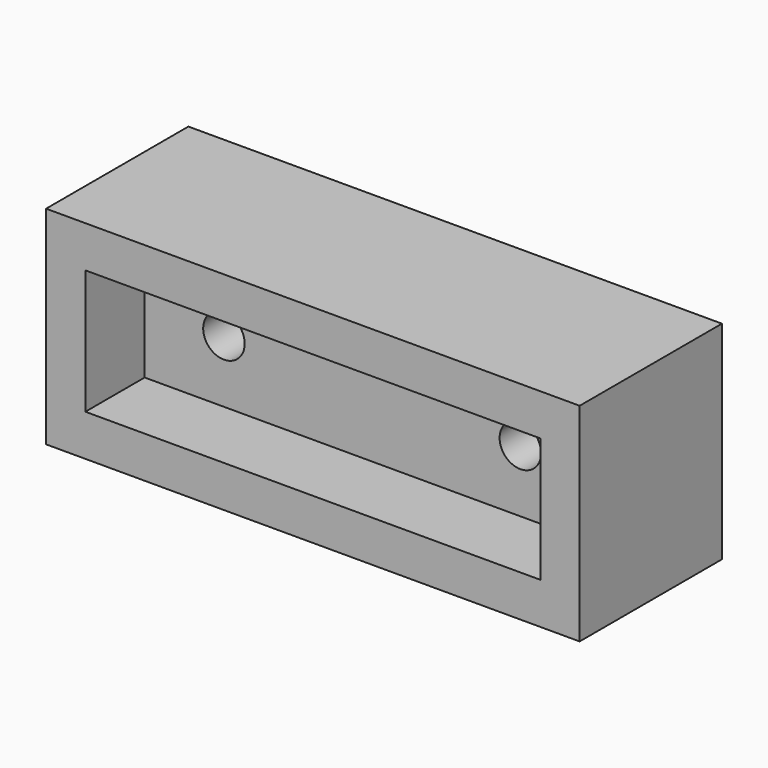
from build123d import *

# Parameters (mm, degrees)
F0_W     = 36
F0_H     = 14
F1_DEPTH = 12
F2_W     = 30.7
F2_H     = 8.4
F3_DEPTH = 5
F4_R     = 1.4
F5_DEPTH = 7


# Not quite as in the source:
# - a pattern or mirror of a feature is missing from the dataset's text; its kind, count and spacing are read off the source's solid


with BuildPart() as f1:
    # F0 (on Front) → F1 (new body)
    with BuildSketch(Plane.XZ):
        Rectangle(F0_W, F0_H)
    extrude(amount=F1_DEPTH)

    # F2 (on face) → F3 (cut)
    with BuildSketch(Plane.XZ.offset(12)):
        Rectangle(F2_W, F2_H)
    extrude(amount=-F3_DEPTH, mode=Mode.SUBTRACT)

    # F4 (on face) → F5 (cut, through all)
    with BuildSketch(Plane.XZ.offset(7)):
        with Locations((-10, 0)):
            Circle(F4_R)
    f5 = extrude(amount=-F5_DEPTH, mode=Mode.SUBTRACT)

    # F5_copies: F5 across plane
    add(f5.mirror(Plane(origin=(0, 0, 0), x_dir=(0, 0, 1), z_dir=(1, 0, 0))), mode=Mode.SUBTRACT)


solid = f1.part
